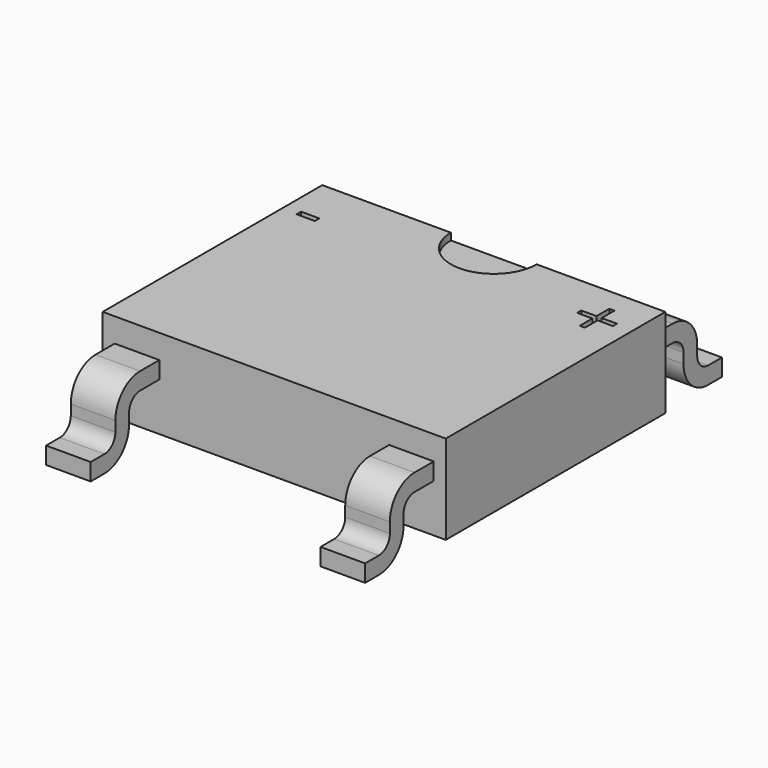
from build123d import *

# Parameters (mm, degrees)
F0_W          = 5
F0_H          = 4
F1_DEPTH      = 1.3
F3_DEPTH      = 2.5
F4_W          = 3.35
F4_H          = 6.5
F4_W_2        = 0.175
F5_DEPTH      = 1.301
F5_DEPTH_BACK = 0.101
F6_R          = 0.625
F6_TEXT_SIZE  = 1.1111111111
F7_DEPTH      = 0.1
F8_R          = 0.2
F8_2_R        = 0.2
F9_R          = 0.45
F9_2_R        = 0.45


# Not quite as in the source:
# - Text() gives the source's letters only with a copy of the font that has no kerning and outlines rounded to 1/6400 em; it was checked with that copy


with BuildPart() as f1:
    # F0 (on Top) → F1 (new body)
    with BuildSketch(Plane.XY):
        Rectangle(F0_W, F0_H)
    extrude(amount=F1_DEPTH)

    # F6 (on face) → F7 (cut)
    with BuildSketch(Plane.XY.offset(1.3)):
        with Locations((0, 2)):
            Circle(F6_R)
        with Locations((1.6751736111, 1)):
            Text('+', F6_TEXT_SIZE, font='Open Sans', text_align=(TextAlign.LEFT, TextAlign.BOTTOM))
        with Locations((-2.325, 1)):
            Text('-', F6_TEXT_SIZE, font='Open Sans', text_align=(TextAlign.LEFT, TextAlign.BOTTOM))
    extrude(amount=-F7_DEPTH, mode=Mode.SUBTRACT)


with BuildPart() as f3:
    # F2 (on Right) → F3 (new body, symmetric)
    with BuildSketch(Plane.YZ):
        Polygon((-3.25, 0.15), (-3.25, -0.1), (-2.55, -0.1), (-2.55, 0.7), (-2, 0.7), (-2, 0.95), (-2.8, 0.95), (-2.8, 0.15), align=None)
    extrude(amount=F3_DEPTH, both=True)


with BuildPart() as f3b:
    # F2 (on Right) → F3, piece 2 (new body, symmetric)
    with BuildSketch(Plane.YZ):
        Polygon((2.8, 0.95), (2, 0.95), (2, 0.7), (2.55, 0.7), (2.55, -0.1), (3.25, -0.1), (3.25, 0.15), (2.8, 0.15), align=None)
    extrude(amount=F3_DEPTH, both=True)


with BuildPart() as f5_tool:
    # F4 (on Top) → F5 (new body, two sides)
    with BuildSketch(Plane.XY) as f5_sk:
        Rectangle(F4_W, F4_H)
        with Locations((2.4125, 0)):
            Rectangle(F4_W_2, F4_H)
        with Locations((-2.4125, 0)):
            Rectangle(F4_W_2, F4_H)
    extrude(amount=F5_DEPTH)
    extrude(f5_sk.sketch, amount=-F5_DEPTH_BACK)


with BuildPart() as f3_1:
    add(f3.part)

    # F5: cut by f5_tool
    add(f5_tool.part, mode=Mode.SUBTRACT)

    # F8
    f8_edges = [f3_1.edges().sort_by_distance(p)[0] for p in [
        (2, -2.8, 0.15),
        (-2, -2.8, 0.15),
        (-2, -2.55, 0.7),
        (2, -2.55, 0.7),
    ]]
    fillet(f8_edges, radius=F8_R)

    # F9
    f9_edges = [f3_1.edges().sort_by_distance(p)[0] for p in [
        (2, -2.8, 0.95),
        (-2, -2.8, 0.95),
        (-2, -2.55, -0.1),
        (2, -2.55, -0.1),
    ]]
    fillet(f9_edges, radius=F9_R)


with BuildPart() as f3b_1:
    add(f3b.part)

    # F5: cut by f5_tool
    add(f5_tool.part, mode=Mode.SUBTRACT)

    # F8#2
    f8_2_edges = [f3b_1.edges().sort_by_distance(p)[0] for p in [
        (-2, 2.8, 0.15),
        (2, 2.8, 0.15),
        (-2, 2.55, 0.7),
        (2, 2.55, 0.7),
    ]]
    fillet(f8_2_edges, radius=F8_2_R)

    # F9#2
    f9_2_edges = [f3b_1.edges().sort_by_distance(p)[0] for p in [
        (2, 2.8, 0.95),
        (-2, 2.8, 0.95),
        (-2, 2.55, -0.1),
        (2, 2.55, -0.1),
    ]]
    fillet(f9_2_edges, radius=F9_2_R)


solid = Compound([f1.part, f3_1.part, f3b_1.part])
